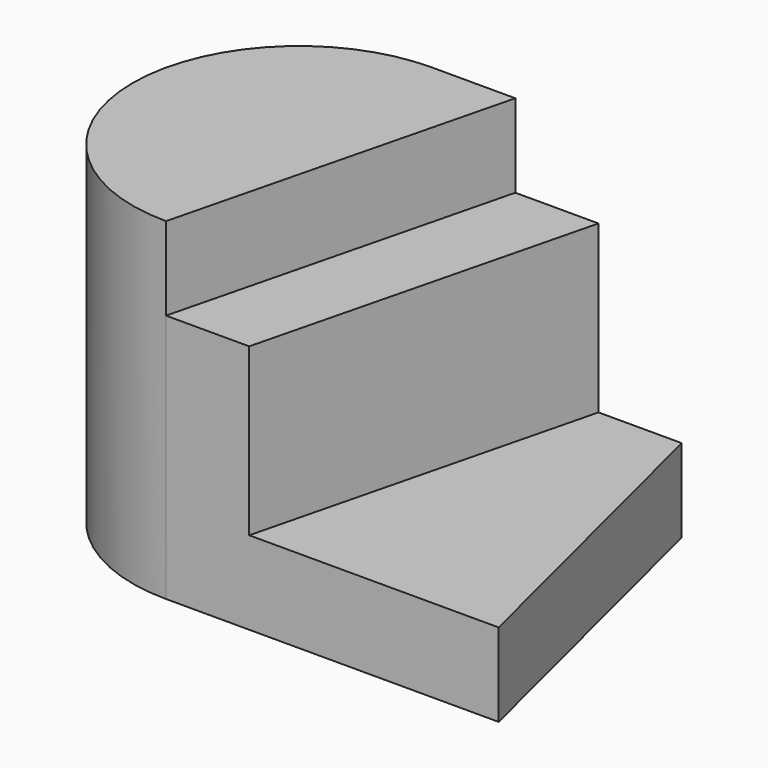
from build123d import *

# Parameters (mm, degrees)
F0_W     = 60
F0_H     = 40
F1_DEPTH = 40
F2_R     = 19.99999
F4_DEPTH = 40
F6_DEPTH = 30
F8_DEPTH = 10


# Not quite as in the source:
# - a fillet or chamfer is up to 0.001 mm smaller than in the source, because OpenCascade refuses the exact size


with BuildPart() as f1:
    # F0 (on Top) → F1 (new body)
    with BuildSketch(Plane.XY):
        with Locations((3.9320588112, -1.0595708795)):
            Rectangle(F0_W, F0_H)
    extrude(amount=F1_DEPTH)

    # F2 (radius 20 in the source; OpenCascade refuses exactly that, so slightly less here)
    f2_edges = [f1.edges().sort_by_distance(p)[0] for p in [
        (-26.067941, 18.940429, 20),
        (-26.067941, -21.059571, 20),
    ]]
    fillet(f2_edges, radius=F2_R)

    # F3 (on face) → F4 (cut)
    with BuildSketch(Plane.XY.offset(40)):
        Polygon((33.9320588112, -21.0595708795), (33.9320588112, 18.9404291205), (23.9320588112, 18.9404291205), align=None)
    extrude(amount=-F4_DEPTH, mode=Mode.SUBTRACT)

    # F5 (on face) → F6 (cut)
    with BuildSketch(Plane.XY.offset(40)):
        Polygon((33.9320588112, -21.0595708795), (23.9320588112, 18.9404291205), (13.9320588112, 18.9404291205), (3.9320588112, -21.0595708795), align=None)
    extrude(amount=-F6_DEPTH, mode=Mode.SUBTRACT)

    # F7 (on face) → F8 (cut)
    with BuildSketch(Plane.XY.offset(40)):
        Polygon((3.9320588112, -21.0595708795), (13.9320588112, 18.9404291205), (3.9320588112, 18.9404291205), (-6.0679411888, -21.0595708795), align=None)
    extrude(amount=-F8_DEPTH, mode=Mode.SUBTRACT)


solid = f1.part
